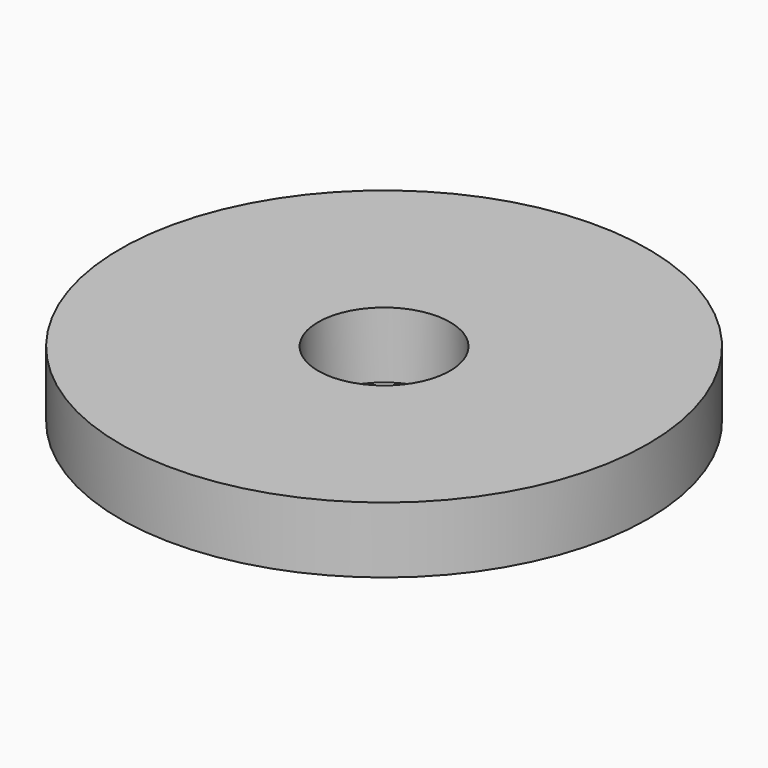
from build123d import *

# Parameters (mm, degrees)
F2_R     = 12.7
F3_DEPTH = 3.175
F4_D     = 6.35


# Not quite as in the source:
# - a variable given as a bare number and used for a length is read in inches; the dataset says mm whatever the document's units were


with BuildPart() as f3:
    # F2 (on Top) → F3 (new body)
    with BuildSketch(Plane.XY):
        Circle(F2_R)
    extrude(amount=F3_DEPTH)

    # F4 (through all)
    with Locations(Plane(origin=(0, 0, 0), x_dir=(1, 0, 0), z_dir=(0, 0, -1))):
        with Locations((0, 0)):
            Hole(F4_D / 2)


solid = f3.part
